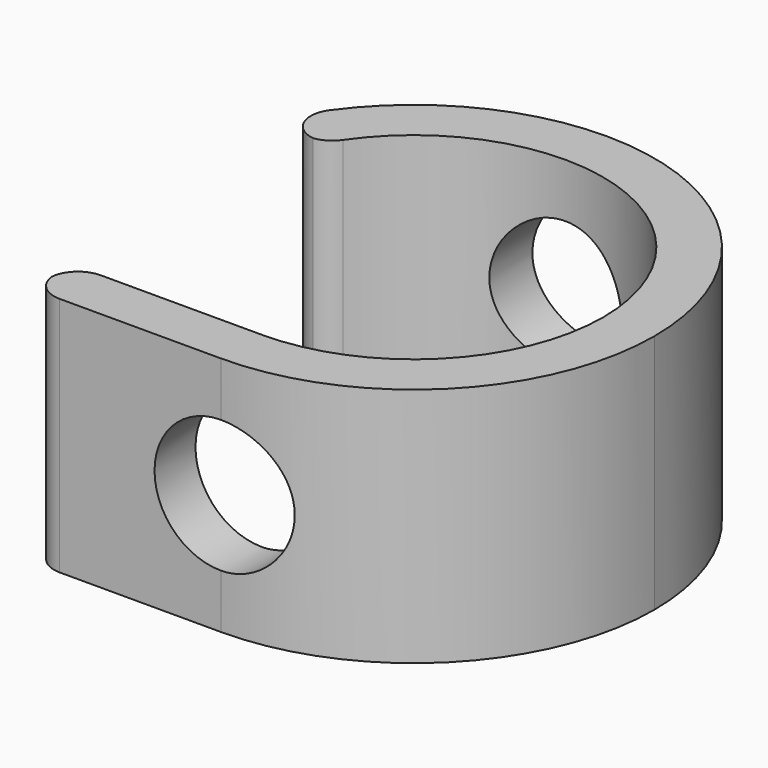
from build123d import *

# Parameters (mm, degrees)
F1_DEPTH      = 12.7
F2_W          = 2.7
F2_H          = 12.7
F3_DEPTH      = 10
F4_R          = 3.5
F5_DEPTH      = 2.701
F5_DEPTH_BACK = 22.701
F6_T1_DEPTH   = 20.2
F7_W          = 8.7146805599
F7_H          = 16.2741800305
F8_DEPTH      = 5
F9_T1_DEPTH   = 16.8328947133
F9_T3_DEPTH   = 26.2954806011


# Not quite as in the source:
# - a fillet or chamfer that OpenCascade refuses, or shapes differently, is made with other operations: its cross-section is extruded or revolved along the edge and cut away or added


with BuildPart() as f1:
    # F0 (on Top) → F1 (new body)
    with BuildSketch(Plane.XY):
        with BuildLine():
            ThreePointArc((0, -12.7), (8.9802561211, -8.9802561211), (12.7, 0))
            ThreePointArc((12.7, 0), (0, 12.7), (-12.7, 0))
            Line((-12.7, 0), (-10, 0))
            ThreePointArc((-10, 0), (0, 10), (10, 0))
            ThreePointArc((10, 0), (7.0710678119, -7.0710678119), (0, -10))
            Line((0, -10), (0, -12.7))
        make_face()
    extrude(amount=F1_DEPTH)

    # F2 (on face) → F3 (join)
    with BuildSketch(Plane(origin=(0, 0, 0), x_dir=(0, -1, 0), z_dir=(-1, 0, 0))):
        with Locations((11.35, 6.35)):
            Rectangle(F2_W, F2_H)
    extrude(amount=F3_DEPTH)

    # F4 (on face) → F5 (cut, two sides)
    with BuildSketch(Plane(origin=(0, -10, 0), x_dir=(-1, 0, 0), z_dir=(0, 1, 0))) as f5_sk:
        with Locations((0, 6.35)):
            Circle(F4_R)
    extrude(amount=-F5_DEPTH, mode=Mode.SUBTRACT)
    extrude(f5_sk.sketch, amount=F5_DEPTH_BACK, mode=Mode.SUBTRACT)

    # F6: fillet of radius 1.5 on 2 edges, made by hand

    # F6_s2 → F6_t1 (cut)
    with BuildSketch(Plane.XY.offset(-3.75)):
        with BuildLine():
            ThreePointArc((-8.5, -10), (-9.5606601718, -10.4393398282), (-10, -11.5))
            Line((-10, -11.5), (-10, -10))
            Line((-10, -10), (-8.5, -10))
        make_face()
        with BuildLine():
            ThreePointArc((-8.5, -12.7), (-9.5606601718, -12.2606601718), (-10, -11.2))
            Line((-10, -11.2), (-10, -12.7))
            Line((-10, -12.7), (-8.5, -12.7))
        make_face()
    extrude(amount=F6_T1_DEPTH, mode=Mode.SUBTRACT)

    # F7 (on face) → F8 (cut)
    with BuildSketch(Plane.XZ):
        with Locations((-12.651483994, 6.0685008066)):
            Rectangle(F7_W, F7_H)
    extrude(amount=-F8_DEPTH, mode=Mode.SUBTRACT)

    # F9: fillet of radius 1.5 on 2 edges, made by hand

    # F9_s2 → F9_t1 (cut)
    with BuildSketch(Plane.XY.offset(-2.0664473567)):
        with BuildLine():
            ThreePointArc((-9.4868329805, 5), (-8.7874543743, 5.1730223946), (-8.249419983, 5.652173913))
            ThreePointArc((-8.249419983, 5.652173913), (-8.4611229501, 5.3300467562), (-8.6602540378, 5))
            Line((-8.6602540378, 5), (-9.4868329805, 5))
        make_face()
    extrude(amount=F9_T1_DEPTH, mode=Mode.SUBTRACT)

    # F9_s4 → F9_t3 (cut)
    with BuildSketch(Plane.XY.offset(-6.7977403006)):
        with BuildLine():
            ThreePointArc((-10.3423983333, 7.3705357143), (-10.4542350586, 5.812905964), (-9.1208552231, 5))
            Line((-9.1208552231, 5), (-11.6743308159, 5))
            ThreePointArc((-11.6743308159, 5), (-11.0719894554, 6.2210167577), (-10.3423983333, 7.3705357143))
        make_face()
    extrude(amount=F9_T3_DEPTH, mode=Mode.SUBTRACT)


solid = f1.part
